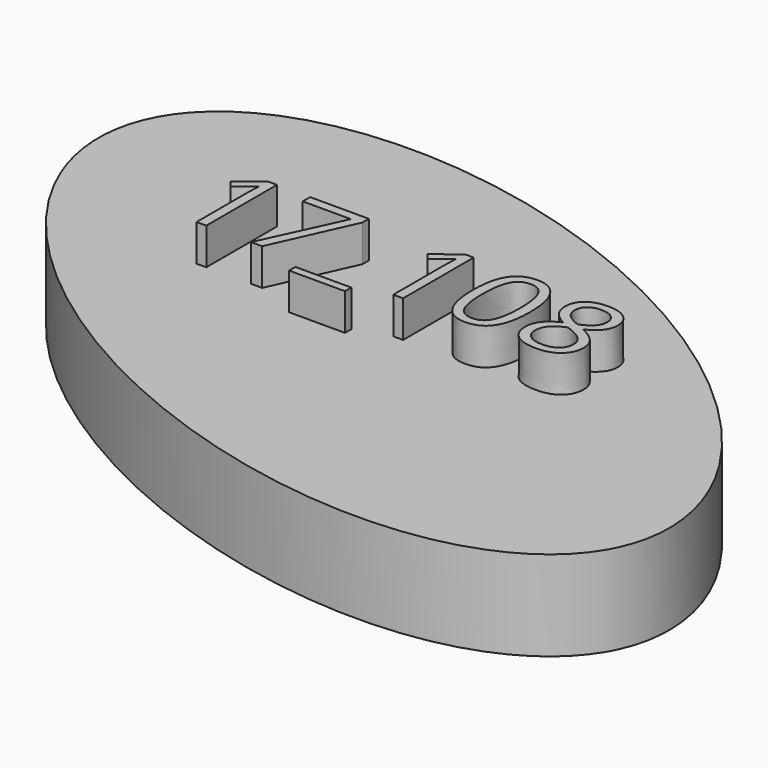
from build123d import *

# Parameters (mm, degrees)
F1_DEPTH     = 18.034
F2_TEXT_SIZE = 24.8029646981
F3_DEPTH     = 25.4


# Not quite as in the source:
# - Text() gives the source's letters only with a copy of the font that has no kerning and outlines rounded to 1/6400 em; it was checked with that copy


with BuildPart() as f1:
    # F0 (on Top) → F1 (new body)
    with BuildSketch(Plane.XY):
        with BuildLine():
            add(Edge.make_bspline(
                [(74.2309316993, -33.6335934699), (104.6743331664, 33.5564335794), (-21.8937651161, 50.4118102595), (-148.4618633986, 67.2671869397), (-52.3371665832, -16.7782167897), (43.7875302321, -100.8236205191), (74.2309316993, -33.6335934699)],
                knots=[0, 0, 0, 2.0943951024, 2.0943951024, 4.1887902048, 4.1887902048, 6.2831853072, 6.2831853072, 6.2831853072], degree=2, weights=[1, 0.5, 1, 0.5, 1, 0.5, 1]))
        make_face()
    extrude(amount=F1_DEPTH)

    # F2 (on Top) → F3 (join)
    with BuildSketch(Plane.XY):
        with Locations((-44.2976698072, 0)):
            Text('17_108', F2_TEXT_SIZE, font='Open Sans', text_align=(TextAlign.LEFT, TextAlign.BOTTOM))
    extrude(amount=F3_DEPTH)


solid = f1.part
